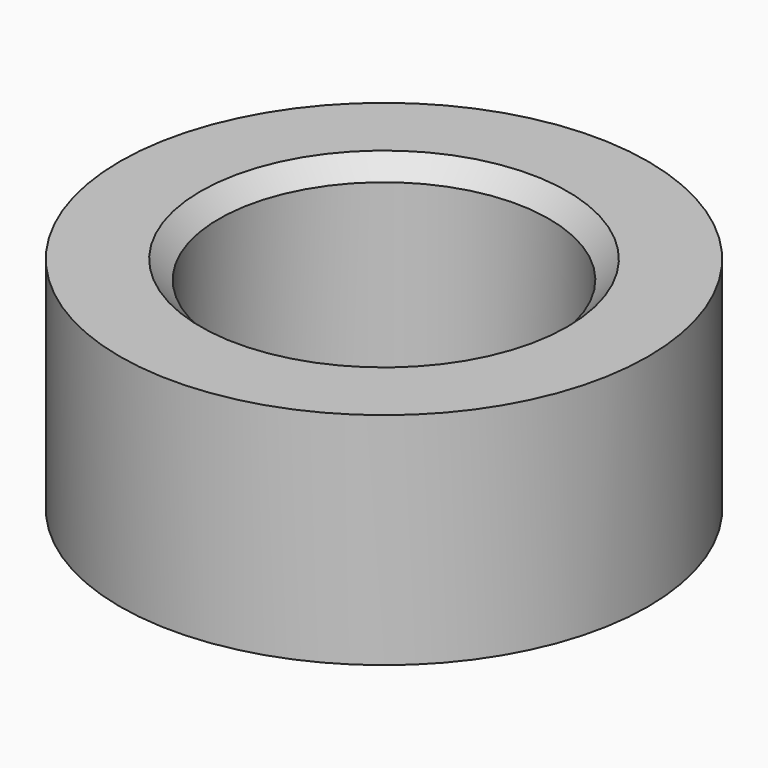
from build123d import *

# Parameters (mm, degrees)
F0_R     = 7.2
F0_R_2   = 4.5
F1_DEPTH = 6
F2_SIZE2 = 0.5
F2_SIZE  = 0.5


# Not quite as in the source:
# - a fillet or chamfer that OpenCascade refuses, or shapes differently, is made with other operations: its cross-section is extruded or revolved along the edge and cut away or added


with BuildPart() as f1:
    # F0 (on Top) → F1 (new body)
    with BuildSketch(Plane.XY):
        Circle(F0_R)
        Circle(F0_R_2, mode=Mode.SUBTRACT)
    extrude(amount=F1_DEPTH)

    # F2
    f2_edges = [f1.edges().sort_by_distance(p)[0] for p in [
        (-4.5, 0, 0),
    ]]
    chamfer(f2_edges, length=F2_SIZE, length2=F2_SIZE2)

    # F3: chamfer of 0.5 on 3 edges, made by hand

    # F3_s1 → F3_t2 (revolve, cut)
    with BuildSketch(Plane.XZ):
        Polygon((4.5, 0.7071067812), (4.6464466094, 0.3535533906), (4.5, 0.5), align=None)
    revolve(axis=Axis((0, 0, 0.5), (0, 0, 1)), mode=Mode.SUBTRACT)

    # F3_s3 → F3_t4 (revolve, cut)
    with BuildSketch(Plane.XZ):
        Polygon((4.5, 5.5), (5, 6), (4.5, 6), align=None)
    revolve(axis=Axis((0, 0, 6), (0, 0, 1)), mode=Mode.SUBTRACT)


solid = f1.part
